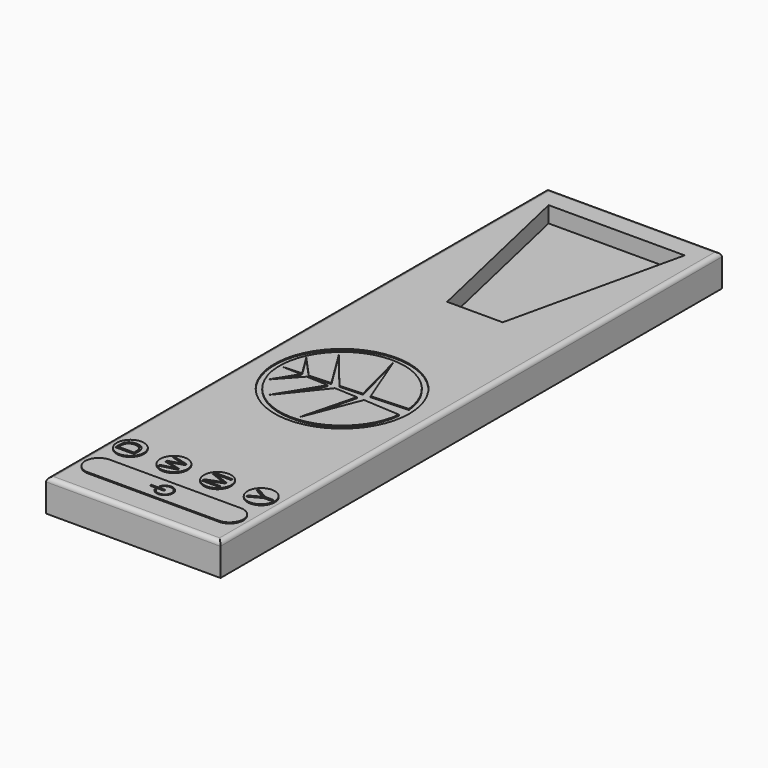
from build123d import *

# Parameters (mm, degrees)
F0_W          = 292.1
F0_H          = 15
F1_DEPTH      = 81.28
F3_DEPTH      = 7.5
F4_R          = 6.35
F5_DEPTH      = 0.5
F6_TEXT_SIZE  = 12.3436676249
F7_DEPTH      = 0.5
F8_TEXT_SIZE  = 10.3328817713
F9_DEPTH      = 0.5
F10_TEXT_SIZE = 11.2017870041
F11_DEPTH     = 0.5
F12_TEXT_SIZE = 13.2963877817
F13_DEPTH     = 0.5
F14_W         = 6.6006779571
F14_H         = 0.8128
F15_DEPTH     = 0.5
F16_R         = 31.4433527127
F17_DEPTH     = 0.5
F18_R         = 2
F19_R         = 9.525
F20_DEPTH     = 2
F21_SIZE      = 1.99999


# Not quite as in the source:
# - a fillet or chamfer is up to 0.001 mm smaller than in the source, because OpenCascade refuses the exact size
# - Text() gives the source's letters only with a copy of the font that has no kerning and outlines rounded to 1/6400 em; it was checked with that copy


with BuildPart() as f1:
    # F0 (on Right) → F1 (new body)
    with BuildSketch(Plane.YZ):
        with Locations((-5.2394010127, -3.6437530771)):
            Rectangle(F0_W, F0_H)
    extrude(amount=F1_DEPTH)

    # F2 (on face) → F3 (cut)
    with BuildSketch(Plane.XY.offset(3.8562469229)):
        Polygon((72.3392, 130.2699234338), (40.64, 130.2699234338), (8.9408, 130.2699234338), (27.686, 47.7131047924), (40.64, 47.7131047924), (53.594, 47.7131047924), align=None)
    extrude(amount=-F3_DEPTH, mode=Mode.SUBTRACT)

    # F4 (on face) → F5 (join)
    with BuildSketch(Plane.XY.offset(3.8562469229)):
        with Locations((10.16, -114.8988327102)):
            Circle(F4_R)
        with Locations((30.48, -114.8988327102)):
            Circle(F4_R)
        with Locations((50.8, -114.8988327102)):
            Circle(F4_R)
        with Locations((71.12, -114.8988327102)):
            Circle(F4_R)
        with BuildLine():
            Line((71.4803109261, -126.9006167143), (10.26959768, -126.9006167143))
            ThreePointArc((10.26959768, -126.9006167143), (3.8132917261, -133.4541068644), (10.6779697007, -139.5785101843))
            Line((10.6779697007, -139.5785101843), (71.5081794227, -139.5785101843))
            ThreePointArc((71.5081794227, -139.5785101843), (77.4699846582, -133.2264276018), (71.4803109261, -126.9006167143))
        make_face()
    extrude(amount=F5_DEPTH)

    # F6 (on face) → F7 (cut)
    with BuildSketch(Plane.XY.offset(4.3562469229)):
        with Locations(Location((14.3564590524, -119.1786915019), (0, 0, 90))):
            Text('D', F6_TEXT_SIZE, font='Open Sans', text_align=(TextAlign.LEFT, TextAlign.BOTTOM))
    extrude(amount=-F7_DEPTH, mode=Mode.SUBTRACT)

    # F8 (on face) → F9 (cut)
    with BuildSketch(Plane.XY.offset(4.3562469229)):
        with Locations(Location((34.342975937, -119.6970400129), (0, 0, 90))):
            Text('W', F8_TEXT_SIZE, font='Open Sans', text_align=(TextAlign.LEFT, TextAlign.BOTTOM))
    extrude(amount=-F9_DEPTH, mode=Mode.SUBTRACT)

    # F10 (on face) → F11 (cut)
    with BuildSketch(Plane.XY.offset(4.3562469229)):
        with Locations(Location((54.6781527936, -119.9637897846), (0, 0, 90))):
            Text('M', F10_TEXT_SIZE, font='Open Sans', text_align=(TextAlign.LEFT, TextAlign.BOTTOM))
    extrude(amount=-F11_DEPTH, mode=Mode.SUBTRACT)

    # F12 (on face) → F13 (cut)
    with BuildSketch(Plane.XY.offset(4.3562469229)):
        with Locations(Location((76.4864645637, -118.698850447), (0, 0, 90))):
            Text('Y', F12_TEXT_SIZE, font='Open Sans', text_align=(TextAlign.LEFT, TextAlign.BOTTOM))
    extrude(amount=-F13_DEPTH, mode=Mode.SUBTRACT)

    # F14 (on face) → F15 (cut)
    with BuildSketch(Plane.XY.offset(4.3562469229)):
        with BuildLine():
            Line((37.8746972178, -134.4631525756), (37.3477385545, -134.6783503514))
            ThreePointArc((37.3477385545, -134.6783503514), (44.6842807533, -133.1662787667), (37.296074315, -131.9311198552))
            Line((37.296074315, -131.9311198552), (37.8307515077, -132.1263525756))
            ThreePointArc((37.8307515077, -132.1263525756), (44.1151753406, -133.1769813264), (37.8746972178, -134.4631525756))
        make_face()
        with Locations((37.5746153245, -133.2947525756)):
            Rectangle(F14_W, F14_H)
    extrude(amount=-F15_DEPTH, mode=Mode.SUBTRACT)

    # F16 (on face) → F17 (cut)
    with BuildSketch(Plane.XY.offset(3.8562469229)):
        with Locations((40.64, -29.6812541783)):
            Circle(F16_R)
        with BuildLine():
            ThreePointArc((69.5485662343, -32.674904491), (11.5770241801, -29.5783930653), (69.5690322928, -26.892305538))
            Line((69.5690322928, -26.892305538), (52.4372432465, -27.7344406649))
            Line((52.4372432465, -27.7344406649), (42.3243588906, -1.924988585))
            Line((42.3243588906, -1.924988585), (48.9795843088, -27.9044063375))
            Line((48.9795843088, -27.9044063375), (38.3467872016, -28.4270751561))
            Line((38.3467872016, -28.4270751561), (22.4652762243, -8.6354289336))
            Line((22.4652762243, -8.6354289336), (34.8041417112, -28.6012184521))
            Line((34.8041417112, -28.6012184521), (24.6709311323, -29.0993294523))
            Line((24.6709311323, -29.0993294523), (15.1280633109, -18.6183236928))
            Line((15.1280633109, -18.6183236928), (21.6957118483, -29.2455801831))
            Line((21.6957118483, -29.2455801831), (12.8326746242, -29.6812541783))
            Line((12.8326746242, -29.6812541783), (21.6957118483, -30.1169281734))
            Line((21.6957118483, -30.1169281734), (15.1280633109, -40.7441846638))
            Line((15.1280633109, -40.7441846638), (24.6709311323, -30.2631789043))
            Line((24.6709311323, -30.2631789043), (34.8041417112, -30.7612899045))
            Line((34.8041417112, -30.7612899045), (22.4652762243, -50.727079423))
            Line((22.4652762243, -50.727079423), (38.3467872016, -30.9354332004))
            Line((38.3467872016, -30.9354332004), (48.9795843088, -31.4581020191))
            Line((48.9795843088, -31.4581020191), (42.3243588906, -57.4375197715))
            Line((42.3243588906, -57.4375197715), (52.4372432465, -31.6280676917))
            Line((52.4372432465, -31.6280676917), (69.5485662343, -32.674904491))
        make_face(mode=Mode.SUBTRACT)
    extrude(amount=-F17_DEPTH, mode=Mode.SUBTRACT)

    # F18
    f18_edges = [f1.edges().sort_by_distance(p)[0] for p in [
        (81.28, -5.239401, 3.856247),
        (40.64, -151.289401, 3.856247),
        (0, -5.239401, 3.856247),
        (40.64, 140.810599, 3.856247),
    ]]
    fillet(f18_edges, radius=F18_R)

    # F19 (on face) → F20 (join)
    with BuildSketch(Plane(origin=(0, 0, -11.1437530771), x_dir=(1, 0, 0), z_dir=(0, 0, -1))):
        with Locations((68.58, 138.5894010127)):
            Circle(F19_R)
        with Locations((12.7, 138.5894010127)):
            Circle(F19_R)
        with Locations((68.58, -128.1105989873)):
            Circle(F19_R)
        with Locations((12.7, -128.1105989873)):
            Circle(F19_R)
    extrude(amount=F20_DEPTH)

    # F21 (size 2 in the source; OpenCascade refuses exactly that, so slightly less here)
    f21_edges = [f1.edges().sort_by_distance(p)[0] for p in [
        (59.055, -138.589401, -13.143753),
        (3.175, -138.589401, -13.143753),
        (59.055, 128.110599, -13.143753),
        (3.175, 128.110599, -13.143753),
    ]]
    chamfer(f21_edges, length=F21_SIZE)


solid = f1.part
